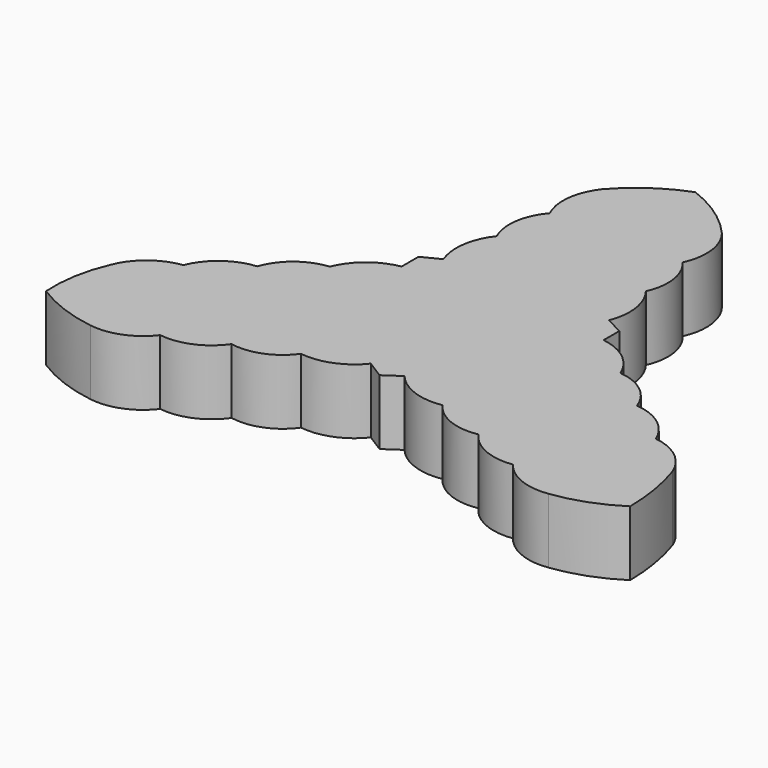
from build123d import *

# Parameters (mm, degrees)
F1_DEPTH = 7.9375


# Not quite as in the source:
# - a length typed as a fraction of an inch, garbled in the dataset ("3 / 203.2 mm" for 3/8 in), is restored


with BuildPart() as f1:
    # F0 (on Top) → F1 (new body)
    with BuildSketch(Plane.XY):
        with BuildLine():
            ThreePointArc((-0.0986067535, 34.0497419238), (-4.0682176485, 31.9659465467), (-7.4162920937, 28.9842672646))
            ThreePointArc((-7.4162920937, 28.9842672646), (-8.8119305122, 25.5953281623), (-8.2258973271, 21.977417171))
            ThreePointArc((-8.2258973271, 21.977417171), (-9.7181261566, 18.698842434), (-9.2097157612, 15.1327075437))
            ThreePointArc((-9.2097157612, 15.1327075437), (-10.6205392688, 11.8246856933), (-10.2093555033, 8.2519613206))
            Line((-10.2093555033, 8.2519613206), (-12.369341217, 7.1464567445))
            Line((-12.369341217, 7.1464567445), (-12.369341217, 4.6386048198))
            Line((-12.369341217, 4.6386048198), (-12.369341217, 4.5682978211))
            ThreePointArc((-12.369341217, 4.5682978211), (-15.5930977879, 3.1185654947), (-17.7027139134, 0.2823972963))
            ThreePointArc((-17.7027139134, 0.2823972963), (-21.0452825194, -1.0603738309), (-23.1384971151, -3.9919692741))
            ThreePointArc((-23.1384971151, -3.9919692741), (-26.5647165348, -5.2934051439), (-28.80180468, -8.19653302))
            ThreePointArc((-28.80180468, -8.19653302), (-32.1117440701, -9.5846599904), (-34.254974256, -12.4637500588))
            ThreePointArc((-34.254974256, -12.4637500588), (-35.4454588739, -16.4293701566), (-35.6585793197, -20.564340055))
            ThreePointArc((-35.6585793197, -20.564340055), (-31.9389059128, -22.4150036937), (-27.9142765499, -23.4461606411))
            ThreePointArc((-27.9142765499, -23.4461606411), (-24.3492963179, -23.0296138883), (-21.4921734029, -20.8571857766))
            ThreePointArc((-21.4921734029, -20.8571857766), (-17.8594468391, -20.3713745504), (-15.0192606046, -18.054899429))
            ThreePointArc((-15.0192606046, -18.054899429), (-11.4338171794, -17.7079201351), (-8.5996589687, -15.484556372))
            ThreePointArc((-8.5996589687, -15.484556372), (-5.0294162563, -15.0523544446), (-2.1409380715, -12.9098966718))
            Line((-2.1409380715, -12.9098966718), (0, -14.2561570176))
            Line((0, -14.2561570176), (1.9696742658, -12.9098966718))
            ThreePointArc((1.9696742658, -12.9098966718), (4.9392756736, -15.0084468105), (8.560301624, -15.3410370587))
            ThreePointArc((8.560301624, -15.3410370587), (11.3944598347, -17.5644008218), (14.9799032599, -17.9113801157))
            ThreePointArc((14.9799032599, -17.9113801157), (17.8200894944, -20.2278552371), (21.4528160582, -20.7136664634))
            ThreePointArc((21.4528160582, -20.7136664634), (24.3099389732, -22.886094575), (27.8749192052, -23.3026413279))
            ThreePointArc((27.8749192052, -23.3026413279), (31.8832272801, -22.3269581873), (35.5659238994, -20.4678624868))
            ThreePointArc((35.5659238994, -20.4678624868), (35.2059818343, -16.3418066269), (34.2156169113, -12.3202307456))
            ThreePointArc((34.2156169113, -12.3202307456), (32.0723867254, -9.4411406771), (28.7624473353, -8.0530137067))
            ThreePointArc((28.7624473353, -8.0530137067), (26.5253591901, -5.1498858306), (23.0991397704, -3.8484499608))
            ThreePointArc((23.0991397704, -3.8484499608), (21.0059251747, -0.9168545176), (17.6633565687, 0.4259166096))
            ThreePointArc((17.6633565687, 0.4259166096), (15.4847616458, 3.3168082822), (12.1560195839, 4.739132713))
            Line((12.1560195839, 4.739132713), (12.1560195839, 7.1464567445))
            Line((12.1560195839, 7.1464567445), (9.9960338703, 8.2519613206))
            ThreePointArc((9.9960338703, 8.2519613206), (10.4072176357, 11.8246856933), (8.9963941282, 15.1327075437))
            ThreePointArc((8.9963941282, 15.1327075437), (9.5048045235, 18.698842434), (8.012575694, 21.977417171))
            ThreePointArc((8.012575694, 21.977417171), (8.5986088792, 25.5953281623), (7.2029704606, 28.9842672646))
            ThreePointArc((7.2029704606, 28.9842672646), (3.8655773676, 31.9687453881), (-0.0986067535, 34.0497419238))
        make_face()
    extrude(amount=F1_DEPTH)


solid = f1.part
